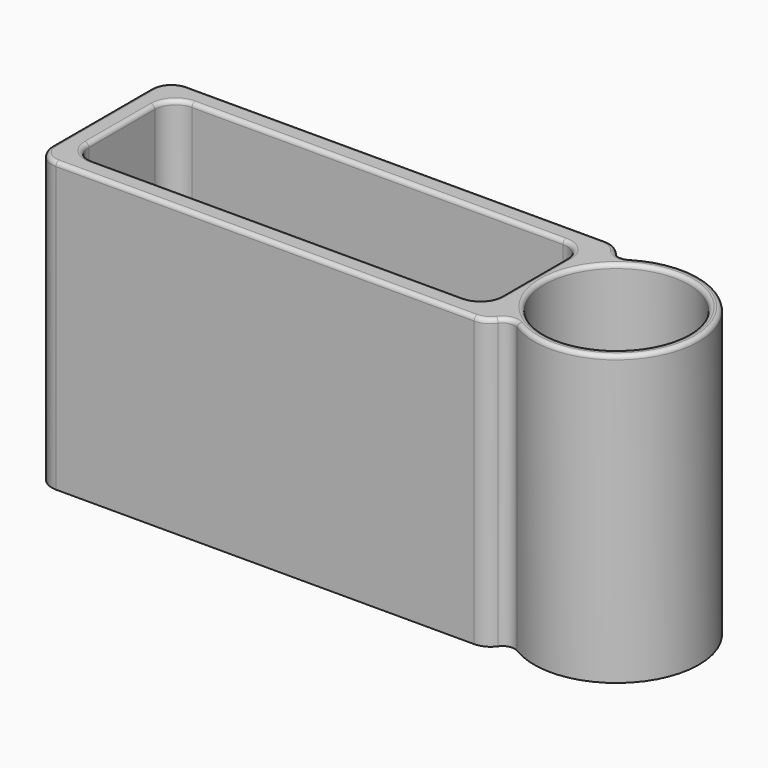
from build123d import *

# Parameters (mm, degrees)
F0_W          = 110
F0_H          = 40
F1_DEPTH      = 70
F2_T          = -5
F3_R          = 20
F4_DEPTH      = 70
F5_R          = 17.5
F6_DEPTH      = 65
F7_R          = 3
F8_R          = 5
F9_R          = 5
F10_R         = 1
F11_TEXT_SIZE = 11.0311543931
F12_DEPTH     = 2
F13_R         = 2
F14_R         = 2


# Not quite as in the source:
# - Text() gives the source's letters only with a copy of the font that has no kerning and outlines rounded to 1/6400 em; it was checked with that copy


with BuildPart() as f1:
    # F0 (on Top) → F1 (new body)
    with BuildSketch(Plane.XY):
        with Locations((-1.2253616005, 37.0818381277)):
            Rectangle(F0_W, F0_H)
    extrude(amount=F1_DEPTH)

    # F2
    f2_openings = [f1.faces().sort_by_distance(p)[0] for p in [
        (-1.225362, 37.081838, 70),
    ]]
    offset(amount=F2_T, openings=f2_openings)

    # F3 (on Top) → F4 (join)
    with BuildSketch(Plane.XY):
        with Locations((68.7746383995, 37.0818381277)):
            Circle(F3_R)
    extrude(amount=F4_DEPTH)

    # F5 (on face) → F6 (cut)
    with BuildSketch(Plane.XY.offset(70)):
        with Locations((68.7746383995, 37.0818381277)):
            Circle(F5_R)
    extrude(amount=-F6_DEPTH, mode=Mode.SUBTRACT)

    # F7
    f7_edges = [f1.edges().sort_by_distance(p)[0] for p in [
        (53.774638, 23.853082, 35),
        (53.774638, 50.310595, 35),
    ]]
    fillet(f7_edges, radius=F7_R)

    # F8
    f8_edges = [f1.edges().sort_by_distance(p)[0] for p in [
        (53.774638, 17.081838, 35),
        (53.774638, 57.081838, 35),
        (-56.225362, 17.081838, 35),
        (-56.225362, 57.081838, 35),
    ]]
    fillet(f8_edges, radius=F8_R)

    # F9
    f9_edges = [f1.edges().sort_by_distance(p)[0] for p in [
        (48.774638, 52.081838, 37.5),
        (-51.225362, 52.081838, 37.5),
        (48.774638, 22.081838, 37.5),
        (-51.225362, 22.081838, 37.5),
    ]]
    fillet(f9_edges, radius=F9_R)

    # F10
    f10_edges = [f1.edges().sort_by_distance(p)[0] for p in [
        (48.774638, 37.081838, 70),
        (47.310172, 50.617372, 70),
        (47.310172, 23.546304, 70),
        (-1.225362, 52.081838, 70),
        (-1.225362, 22.081838, 70),
        (-49.760896, 50.617372, 70),
        (-49.760896, 23.546304, 70),
        (-51.225362, 37.081838, 70),
        (56.169771, 20.398811, 70),
        (52.542131, 17.641009, 70),
        (88.774638, 37.081838, 70),
        (-0.490423, 17.081838, 70),
        (56.169771, 53.764865, 70),
        (-54.760896, 18.546304, 70),
        (52.542131, 56.522667, 70),
        (-56.225362, 37.081838, 70),
        (-0.490423, 57.081838, 70),
        (-54.760896, 55.617372, 70),
        (51.274638, 37.081838, 70),
    ]]
    fillet(f10_edges, radius=F10_R)

    # F11 (on face) → F12 (cut)
    with BuildSketch(Plane(origin=(0, 57.0818381277, 0), x_dir=(-1, 0, 0), z_dir=(0, 1, 0))):
        with Locations((-40.8049581953, 54.8973690322)):
            Text('3D Design by AJ', F11_TEXT_SIZE, font='Open Sans', text_align=(TextAlign.LEFT, TextAlign.BOTTOM))
    extrude(amount=-F12_DEPTH, mode=Mode.SUBTRACT)

    # F13
    f13_edges = [f1.edges().sort_by_distance(p)[0] for p in [
        (-1.225362, 22.081838, 5),
        (-49.760896, 23.546304, 5),
        (47.310172, 23.546304, 5),
        (-51.225362, 37.081838, 5),
        (48.774638, 37.081838, 5),
        (-49.760896, 50.617372, 5),
        (47.310172, 50.617372, 5),
        (-1.225362, 52.081838, 5),
    ]]
    fillet(f13_edges, radius=F13_R)

    # F14
    f14_edges = [f1.edges().sort_by_distance(p)[0] for p in [
        (51.274638, 37.081838, 5),
    ]]
    fillet(f14_edges, radius=F14_R)


solid = f1.part
